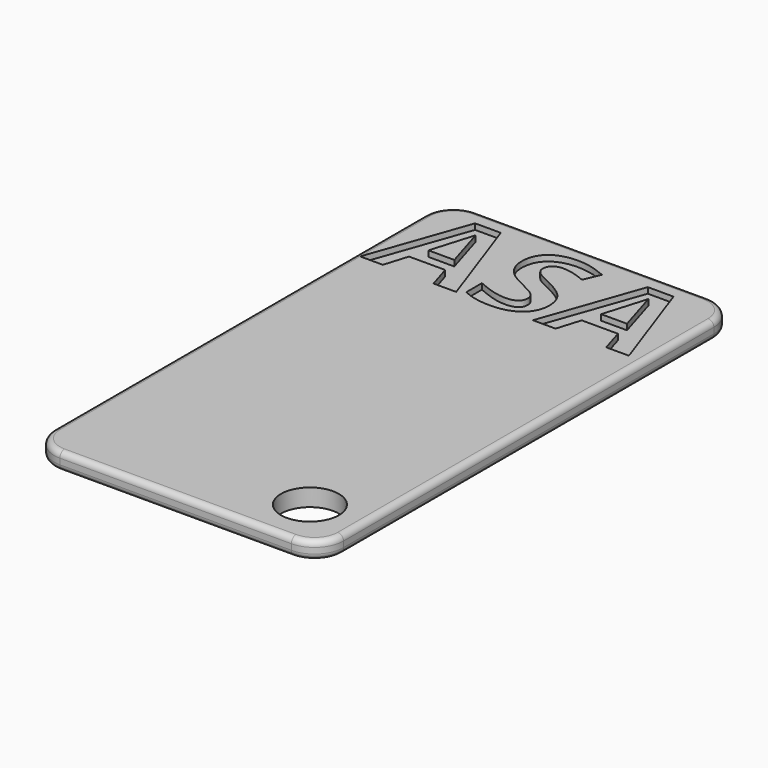
from build123d import *

# Parameters (mm, degrees)
F0_W         = 90
F0_H         = 50
F1_DEPTH     = 3
F2_R         = 1
F3_T1_DEPTH  = 3
F3_T4_ANGLE  = 90
F3_T6_ANGLE  = 90
F3_T8_ANGLE  = 90
F3_T10_ANGLE = 90
F3_T12_ANGLE = 90
F3_T14_ANGLE = 90
F3_T16_ANGLE = 90
F3_T18_ANGLE = 90
F5_ANGLE     = 90
F6_TEXT_SIZE = 24.0526150955
F7_DEPTH     = 1
F8_R         = 5
F9_DEPTH     = 3


# Not quite as in the source:
# - a fillet or chamfer that OpenCascade refuses, or shapes differently, is made with other operations: its cross-section is extruded or revolved along the edge and cut away or added
# - Text() gives the source's letters only with a copy of the font that has no kerning and outlines rounded to 1/6400 em; it was checked with that copy


with BuildPart() as f1:
    # F0 (on Top) → F1 (new body)
    with BuildSketch(Plane.XY):
        Rectangle(F0_W, F0_H)
    extrude(amount=F1_DEPTH)

    # F2
    f2_edges = [f1.edges().sort_by_distance(p)[0] for p in [
        (0, 25, 3),
        (-45, 0, 3),
        (0, -25, 3),
        (45, 0, 3),
        (0, 25, 0),
        (-45, 0, 0),
        (0, -25, 0),
        (45, 0, 0),
    ]]
    fillet(f2_edges, radius=F2_R)

    # F3: fillet of radius 5 on 4 edges, made by hand

    # F3_s2 → F3_t1 (cut)
    with BuildSketch(Plane.XY):
        with BuildLine():
            ThreePointArc((45, -20), (43.5355339059, -23.5355339059), (40, -25))
            Line((40, -25), (45, -25))
            Line((45, -25), (45, -20))
        make_face()
        with BuildLine():
            ThreePointArc((40, 25), (43.5355339059, 23.5355339059), (45, 20))
            Line((45, 20), (45, 25))
            Line((45, 25), (40, 25))
        make_face()
        with BuildLine():
            ThreePointArc((-40, 25), (-43.5355339059, 23.5355339059), (-45, 20))
            Line((-45, 20), (-45, 25))
            Line((-45, 25), (-40, 25))
        make_face()
        with BuildLine():
            ThreePointArc((-45, -20), (-43.5355339059, -23.5355339059), (-40, -25))
            Line((-40, -25), (-45, -25))
            Line((-45, -25), (-45, -20))
        make_face()
    extrude(amount=F3_T1_DEPTH, mode=Mode.SUBTRACT)

    # F3_s3 → F3_t4 (revolve, cut)
    with BuildSketch(Plane.YZ.offset(-40)):
        with BuildLine():
            ThreePointArc((-24, 0), (-24.7071067812, 0.2928932188), (-25, 1))
            Line((-25, 1), (-25, 0))
            Line((-25, 0), (-24, 0))
        make_face()
    revolve(axis=Axis((-40, -20, 0), (0, 0, -1)), revolution_arc=F3_T4_ANGLE, mode=Mode.SUBTRACT)

    # F3_s5 → F3_t6 (revolve, cut)
    with BuildSketch(Plane.XZ.offset(20)):
        with BuildLine():
            ThreePointArc((-44, 3), (-44.7071067812, 2.7071067812), (-45, 2))
            Line((-45, 2), (-45, 3))
            Line((-45, 3), (-44, 3))
        make_face()
    revolve(axis=Axis((-40, -20, 3), (0, 0, 1)), revolution_arc=F3_T6_ANGLE, mode=Mode.SUBTRACT)

    # F3_s7 → F3_t8 (revolve, cut)
    with BuildSketch(Plane.XZ.offset(-20)):
        with BuildLine():
            ThreePointArc((-44, 0), (-44.7071067812, 0.2928932188), (-45, 1))
            Line((-45, 1), (-45, 0))
            Line((-45, 0), (-44, 0))
        make_face()
    revolve(axis=Axis((-40, 20, 0), (0, 0, -1)), revolution_arc=F3_T8_ANGLE, mode=Mode.SUBTRACT)

    # F3_s9 → F3_t10 (revolve, cut)
    with BuildSketch(Plane.YZ.offset(-40)):
        with BuildLine():
            ThreePointArc((24, 3), (24.7071067812, 2.7071067812), (25, 2))
            Line((25, 2), (25, 3))
            Line((25, 3), (24, 3))
        make_face()
    revolve(axis=Axis((-40, 20, 3), (0, 0, 1)), revolution_arc=F3_T10_ANGLE, mode=Mode.SUBTRACT)

    # F3_s11 → F3_t12 (revolve, cut)
    with BuildSketch(Plane.YZ.offset(40)):
        with BuildLine():
            ThreePointArc((24, 0), (24.7071067812, 0.2928932188), (25, 1))
            Line((25, 1), (25, 0))
            Line((25, 0), (24, 0))
        make_face()
    revolve(axis=Axis((40, 20, 0), (0, 0, -1)), revolution_arc=F3_T12_ANGLE, mode=Mode.SUBTRACT)

    # F3_s13 → F3_t14 (revolve, cut)
    with BuildSketch(Plane.XZ.offset(-20)):
        with BuildLine():
            ThreePointArc((44, 3), (44.7071067812, 2.7071067812), (45, 2))
            Line((45, 2), (45, 3))
            Line((45, 3), (44, 3))
        make_face()
    revolve(axis=Axis((40, 20, 3), (0, 0, 1)), revolution_arc=F3_T14_ANGLE, mode=Mode.SUBTRACT)

    # F3_s15 → F3_t16 (revolve, cut)
    with BuildSketch(Plane.XZ.offset(20)):
        with BuildLine():
            ThreePointArc((44, 0), (44.7071067812, 0.2928932188), (45, 1))
            Line((45, 1), (45, 0))
            Line((45, 0), (44, 0))
        make_face()
    revolve(axis=Axis((40, -20, 0), (0, 0, -1)), revolution_arc=F3_T16_ANGLE, mode=Mode.SUBTRACT)

    # F3_s17 → F3_t18 (revolve, cut)
    with BuildSketch(Plane.YZ.offset(40)):
        with BuildLine():
            ThreePointArc((-24, 3), (-24.7071067812, 2.7071067812), (-25, 2))
            Line((-25, 2), (-25, 3))
            Line((-25, 3), (-24, 3))
        make_face()
    revolve(axis=Axis((40, -20, 3), (0, 0, 1)), revolution_arc=F3_T18_ANGLE, mode=Mode.SUBTRACT)


with BuildPart() as f1_1:
    # F5: moved
    add(f1.part.rotate(Axis((0, 0, 16.4477843791), (0, 0, 1)), F5_ANGLE))

    # F6 (on face) → F7 (cut)
    with BuildSketch(Plane.XY.offset(3)):
        with Locations((-24, 24.8506928672)):
            Text('ASA', F6_TEXT_SIZE, font='Open Sans', font_style=FontStyle.BOLD, text_align=(TextAlign.LEFT, TextAlign.BOTTOM))
    extrude(amount=-F7_DEPTH, mode=Mode.SUBTRACT)

    # F8 (on face) → F9 (cut)
    with BuildSketch(Plane.XY.offset(3)):
        with Locations((16, -36)):
            Circle(F8_R)
    extrude(amount=-F9_DEPTH, mode=Mode.SUBTRACT)


solid = f1_1.part
